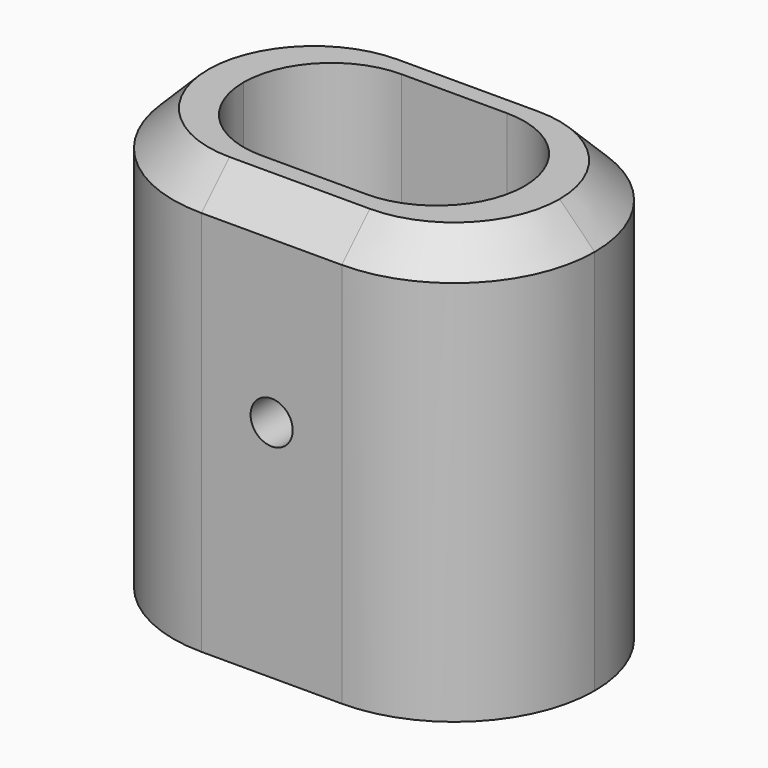
from build123d import *

# Parameters (mm, degrees)
F1_DEPTH = 60
F2_SIZE  = 5
F3_R     = 3
F4_DEPTH = 40.001


with BuildPart() as f1:
    # F0 (on Top) → F1 (new body)
    with BuildSketch(Plane.XY):
        with BuildLine():
            ThreePointArc((30, 0), (24.1421356237, 14.1421356237), (10, 20))
            Line((10, 20), (-10, 20))
            ThreePointArc((-10, 20), (-24.1421356237, 14.1421356237), (-30, 0))
            ThreePointArc((-30, 0), (-24.1421356237, -14.1421356237), (-10, -20))
            Line((-10, -20), (10, -20))
            ThreePointArc((10, -20), (24.1421356237, -14.1421356237), (30, 0))
        make_face()
        with BuildLine():
            Line((-7.5, 12.5), (7.5, 12.5))
            ThreePointArc((7.5, 12.5), (16.3388347648, 8.8388347648), (20, 0))
            ThreePointArc((20, 0), (16.3388347648, -8.8388347648), (7.5, -12.5))
            Line((7.5, -12.5), (-7.5, -12.5))
            ThreePointArc((-7.5, -12.5), (-16.3388347648, -8.8388347648), (-20, 0))
            ThreePointArc((-20, 0), (-16.3388347648, 8.8388347648), (-7.5, 12.5))
        make_face(mode=Mode.SUBTRACT)
    extrude(amount=F1_DEPTH)

    # F2
    f2_edges = [f1.edges().sort_by_distance(p)[0] for p in [
        (30, 0, 60),
        (0, 20, 60),
        (-30, 0, 60),
        (0, -20, 60),
    ]]
    chamfer(f2_edges, length=F2_SIZE)

    # F3 (on face) → F4 (cut, through all)
    with BuildSketch(Plane.XZ.offset(20)):
        with Locations((0, 32)):
            Circle(F3_R)
    extrude(amount=-F4_DEPTH, mode=Mode.SUBTRACT)


solid = f1.part
